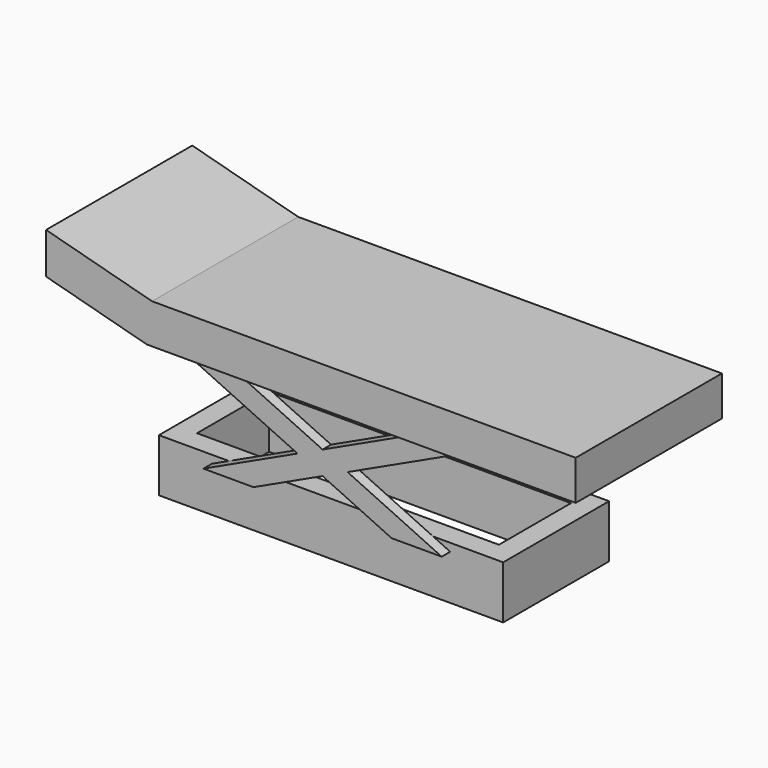
from build123d import *

# Parameters (mm, degrees)
F0_W     = 1300
F0_H     = 500
F0_W_2   = 1140
F0_H_2   = 340
F1_DEPTH = 200
F3_DEPTH = 345
F5_DEPTH = 40
F7_DEPTH = 35


# Not quite as in the source:
# - a feature names something its author has since deleted; it is built from what else it names


with BuildPart() as f1:
    # F0 (on Top) → F1 (new body)
    with BuildSketch(Plane.XY):
        Rectangle(F0_W, F0_H)
        Rectangle(F0_W_2, F0_H_2, mode=Mode.SUBTRACT)
    extrude(amount=F1_DEPTH)



with BuildPart() as f3:
    # F2 (on Front) → F3 (new body, symmetric)
    with BuildSketch(Plane.XZ):
        Polygon((1000, 700), (-600, 700), (-1000, 807.1796769724), (-1000, 651.8882499109), (-619.7478746381, 550), (1000, 550), align=None)
    extrude(amount=F3_DEPTH, both=True)


with BuildPart() as f1_1:
    add(f1.part)

    add(f3.part)  # F5 merges F3
    # F4 (on face) → F5 (join)
    with BuildSketch(Plane.XZ.offset(250)):
        Polygon((-385.6647923847, 200), (-450, 170), (-260.7038733478, 170), (-196.3686657325, 200), align=None)
        Polygon((-94.6480633261, 335.7033294112), (-385.6647923847, 200), (-196.3686657325, 200), (0, 291.5682126528), align=None)
        Polygon((-554.2087564458, 550), (-94.6480633261, 335.7033294112), (0, 379.8384461697), (-364.9126297936, 550), align=None)
        Polygon((0, 379.8384461697), (-94.6480633261, 335.7033294112), (0, 291.5682126528), (94.6480633261, 335.7033294112), align=None)
        Polygon((364.9126297936, 550), (0, 379.8384461697), (94.6480633261, 335.7033294112), (554.2087564458, 550), align=None)
        Polygon((94.6480633261, 335.7033294112), (0, 291.5682126528), (196.3686657325, 200), (385.6647923847, 200), align=None)
        Polygon((385.6647923847, 200), (196.3686657325, 200), (260.7038733478, 170), (450, 170), align=None)
    extrude(amount=F5_DEPTH)

    # F6 (on face) → F7 (join)
    with BuildSketch(Plane(origin=(0, 250, 0), x_dir=(-1, 0, 0), z_dir=(0, 1, 0))):
        Polygon((-554.2087564458, 550), (-94.6480633261, 335.7033294113), (0, 379.8384461697), (-364.9126297936, 550), align=None)
        Polygon((364.9126297936, 550), (0, 379.8384461697), (94.6480633261, 335.7033294113), (554.2087564458, 550), align=None)
        Polygon((0, 379.8384461697), (-94.6480633261, 335.7033294113), (0, 291.5682126528), (94.6480633261, 335.7033294113), align=None)
        Polygon((-94.6480633261, 335.7033294113), (-385.6647923847, 200), (-196.3686657325, 200), (0, 291.5682126528), align=None)
        Polygon((94.6480633261, 335.7033294113), (0, 291.5682126528), (196.3686657325, 200), (385.6647923847, 200), align=None)
        Polygon((385.6647923847, 200), (196.3686657325, 200), (260.7038733478, 170), (450, 170), align=None)
        Polygon((-385.6647923847, 200), (-450, 170), (-260.7038733478, 170), (-196.3686657325, 200), align=None)
    extrude(amount=F7_DEPTH)


solid = f1_1.part
